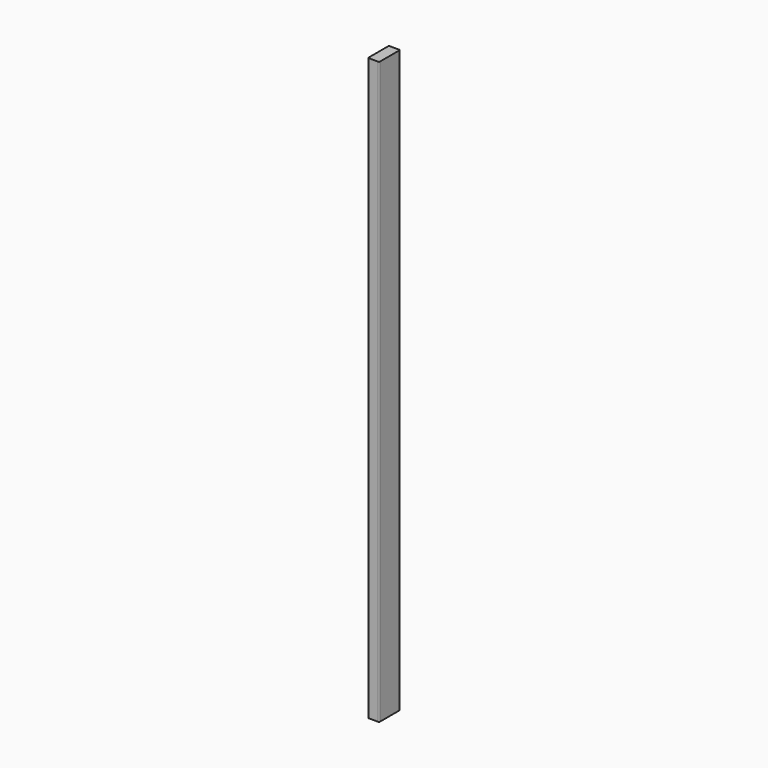
from build123d import *

# Parameters (mm, degrees)
F2_DEPTH = 1981.2


# Not quite as in the source:
# - a variable given as a bare number and used for a length is read in inches; the dataset says mm whatever the document's units were


with BuildPart() as f2:
    # F0 (on Top) → F2 (new body)
    with BuildSketch(Plane.XY):
        with BuildLine():
            ThreePointArc((0, 3.175), (0.9299359697, 0.9299359697), (3.175, 0))
            Line((3.175, 0), (34.925, 0))
            ThreePointArc((34.925, 0), (37.1700640303, 0.9299359697), (38.1, 3.175))
            Line((38.1, 3.175), (38.1, 85.725))
            ThreePointArc((38.1, 85.725), (37.1700640303, 87.9700640303), (34.925, 88.9))
            Line((34.925, 88.9), (3.175, 88.9))
            ThreePointArc((3.175, 88.9), (0.9299359697, 87.9700640303), (0, 85.725))
            Line((0, 85.725), (0, 3.175))
        make_face()
    extrude(amount=F2_DEPTH)


solid = f2.part
